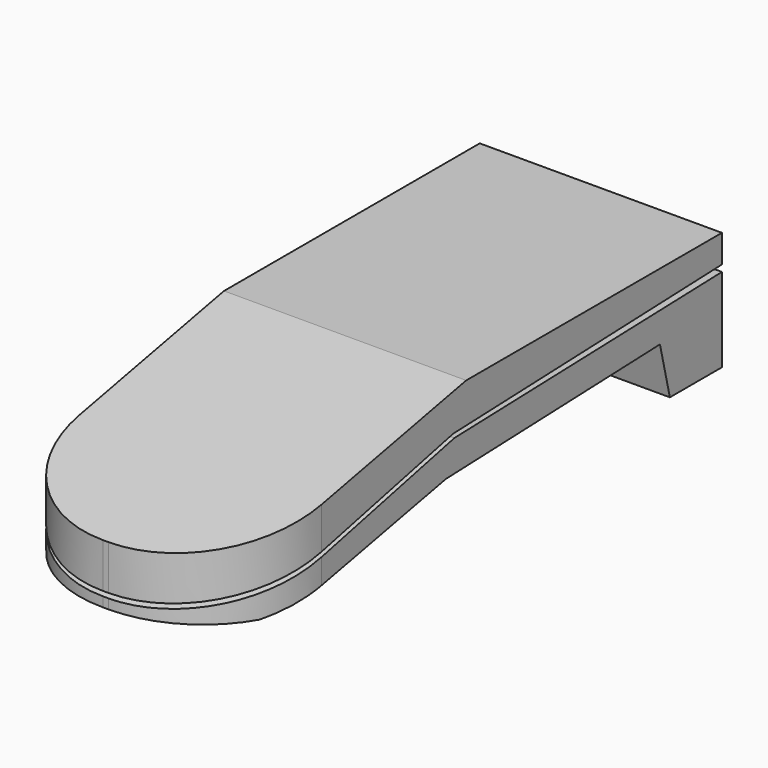
from build123d import *

# Parameters (mm, degrees)
F1_DEPTH    = 57.15
F2_R        = 27.94
F3_T        = -3.048
F4_DEPTH    = 57.15
F5_T1_DEPTH = 141.9948617116
F6_T        = -2.54


# Not quite as in the source:
# - a fillet or chamfer that OpenCascade refuses, or shapes differently, is made with other operations: its cross-section is extruded or revolved along the edge and cut away or added


with BuildPart() as f1:
    # F0 (on Right) → F1 (new body)
    with BuildSketch(Plane.YZ):
        Polygon((-73.1163992389, 13.97), (-73.1163992389, 3.4139757045), (-6.3229924999, 18.4347908944), (72.9336007611, 21.3625766337), (72.9336007611, 27.94), (-2.5041415356, 27.94), align=None)
    extrude(amount=F1_DEPTH)

    # F2
    f2_edges = [f1.edges().sort_by_distance(p)[0] for p in [
        (0, -73.116399, 8.691988),
        (57.15, -73.116399, 8.691988),
    ]]
    fillet(f2_edges, radius=F2_R)

    # F3
    f3_openings = [f1.faces().sort_by_distance(p)[0] for p in [
        (28.575, 33.305304, 19.898684),
        (28.575, -37.106773, 11.51199),
    ]]
    offset(amount=F3_T, openings=f3_openings)


with BuildPart() as f4:
    # F0 (on Right) → F4 (new body)
    with BuildSketch(Plane.YZ):
        Polygon((-73.1163992389, 2.2948617116), (-73.1163992389, 0), (-58.8958412409, 0), (-8.487008512, 9.9060228094), (54.6513311565, 12.197333388), (57.5791150331, 0), (72.9336007611, 0), (72.9336007611, 19.8148395866), (-5.9758147364, 17.3937518685), align=None)
    extrude(amount=F4_DEPTH)

    # F5: fillet of radius 27.94 on 2 edges, made by hand

    # F5_s2 → F5_t1 (cut)
    with BuildSketch(Plane.XY.offset(-69.85)):
        with BuildLine():
            ThreePointArc((29.21, -73.1163992389), (48.9665634664, -64.9329627053), (57.15, -45.1763992389))
            Line((57.15, -45.1763992389), (57.15, -73.1163992389))
            Line((57.15, -73.1163992389), (29.21, -73.1163992389))
        make_face()
        with BuildLine():
            ThreePointArc((27.94, -73.1163992389), (8.1834365336, -64.9329627053), (0, -45.1763992389))
            Line((0, -45.1763992389), (0, -73.1163992389))
            Line((0, -73.1163992389), (27.94, -73.1163992389))
        make_face()
    extrude(amount=F5_T1_DEPTH, mode=Mode.SUBTRACT)

    # F6
    f6_openings = [f4.faces().sort_by_distance(p)[0] for p in [
        (28.575, -36.93138, 10.432319),
        (28.575, 33.478893, 18.604296),
    ]]
    offset(amount=F6_T, openings=f6_openings, kind=Kind.INTERSECTION)


solid = Compound([f1.part, f4.part])
